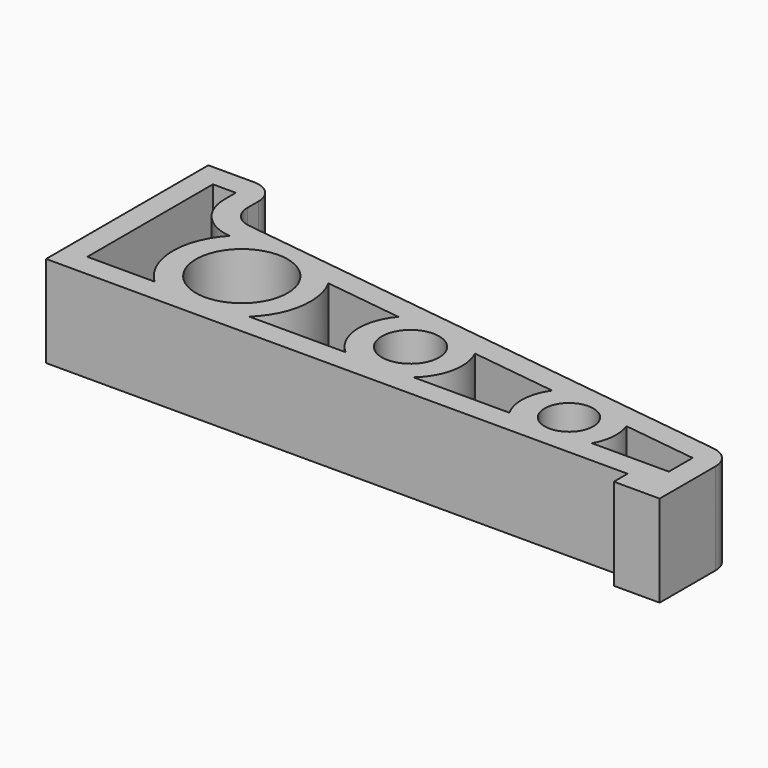
from build123d import *

# Parameters (mm, degrees)
F1_DEPTH    = 8
F2_R        = 2
F3_R        = 4
F3_R_2      = 2.5
F3_R_3      = 2.125
F4_DEPTH    = 8.001
F5_T        = 2
F5_T3_DEPTH = 12


# Not quite as in the source:
# - a shell that OpenCascade refuses in one call is made with other operations: the cavity is built on its own and cut out


with BuildPart() as f1:
    # F0 (on Top) → F1 (new body)
    with BuildSketch(Plane.XY):
        Polygon((-27.375, -6.35), (23.375, -6.35), (23.375, -7.85), (27.375, -7.85), (27.375, -6.35), (27.375, 0), (-21.375, 6.35), (-21.375, 11.35), (-27.375, 11.35), (-27.375, 6.35), align=None)
    extrude(amount=F1_DEPTH)

    # F2
    f2_edges = [f1.edges().sort_by_distance(p)[0] for p in [
        (-21.375, 11.35, 4),
        (27.375, 0, 4),
        (-21.375, 6.35, 4),
    ]]
    fillet(f2_edges, radius=F2_R)

    # F3 (on face) → F4 (cut, through all)
    with BuildSketch(Plane.XY.offset(8)):
        with Locations((-15.375, 0)):
            Circle(F3_R)
        with Locations((0.125, -0.9643055964)):
            Circle(F3_R_2)
        with Locations((15.0608578937, -2.35)):
            Circle(F3_R_3)
    extrude(amount=-F4_DEPTH, mode=Mode.SUBTRACT)

    # F5: shell of thickness 2, made by hand


with BuildPart() as f5_core1:
    # F5_t2: copy of F1
    add(f1.part)

    # the walls: a layer under each face that stays
    f5_faces = [f5_core1.faces().sort_by_distance(p)[0] for p in [
        (27.375, -4.8031912743, 4),
        (25.375, -7.85, 4),
        (3, 3.175, 4),
        (23.375, -7.1, 4),
        (-20.8777742764, 6.7866592918, 4),
        (-2, -6.35, 4),
        (-21.375, 8.7281912743, 4),
        (-27.375, 2.5, 4),
        (-25.375, 11.35, 4),
        (-2.375, -0.9643055964, 4),
        (12.9358578937, -2.35, 4),
        (-19.375, 0, 4),
        (0, 1.75, 0),
    ]]
    thicken(f5_faces, amount=-F5_T, mode=Mode.SUBTRACT)

    # F5_s4 → F5_t3 (cut)
    with BuildSketch(Plane.XY.offset(-2)):
        Polygon((23.355, -6.37), (25.375, -6.35), (25.375, -4.35), (23.375, -4.35), align=None)
    extrude(amount=F5_T3_DEPTH, mode=Mode.SUBTRACT)


with BuildPart() as f1_1:
    add(f1.part)

    # what is left inside the walls is the cavity
    f5_cavity = [f5_core1.part.solids().sort_by_distance(p)[0] for p in [
        (22.021788, -4.33, 6),
        (7.27122, -4.33, 6),
        (-25.355, 2.5, 6),
        (-7.040903, -4.33, 6),
    ]]
    add(f5_cavity, mode=Mode.SUBTRACT)


solid = f1_1.part
